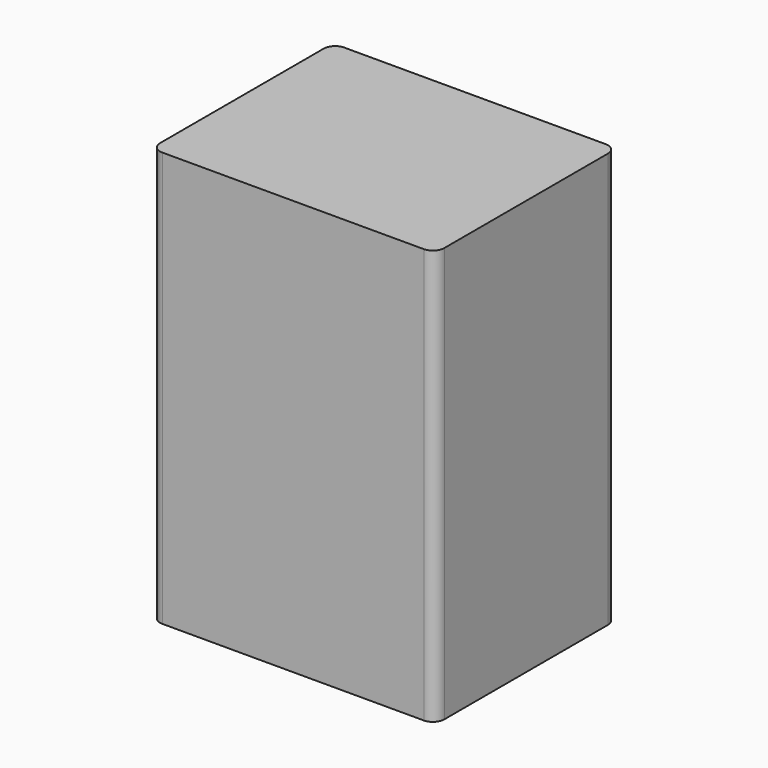
from build123d import *

# Parameters (mm, degrees)
F1_DEPTH = 2190
F2_T     = -2.54


# Not quite as in the source:
# - a shell that OpenCascade refuses in one call is made with other operations: the cavity is built on its own and cut out


with BuildPart() as f1:
    # F0 (on Top) → F1 (new body)
    with BuildSketch(Plane.XY):
        with BuildLine():
            Line((690, 600), (-690, 600))
            ThreePointArc((-690, 600), (-732.4264068712, 582.4264068712), (-750, 540))
            Line((-750, 540), (-750, -540))
            ThreePointArc((-750, -540), (-732.4264068712, -582.4264068712), (-690, -600))
            Line((-690, -600), (690, -600))
            ThreePointArc((690, -600), (732.4264068712, -582.4264068712), (750, -540))
            Line((750, -540), (750, 540))
            ThreePointArc((750, 540), (732.4264068712, 582.4264068712), (690, 600))
        make_face()
    extrude(amount=F1_DEPTH)

    # F2: a shell. OpenCascade refuses it in one call, so the cavity is built on its own and cut out:
    # the body offset inwards by the wall thickness, plus a prism from it out through each open face.
    f2_core = offset(f1.part, amount=F2_T, mode=Mode.PRIVATE)
    f2_exits = [f2_core.faces().sort_by_distance(p)[0] for p in [
        (0, 597.46, 1095),
    ]]
    add(f2_core, mode=Mode.SUBTRACT)
    extrude(f2_exits, amount=-F2_T, mode=Mode.SUBTRACT)


solid = f1.part
